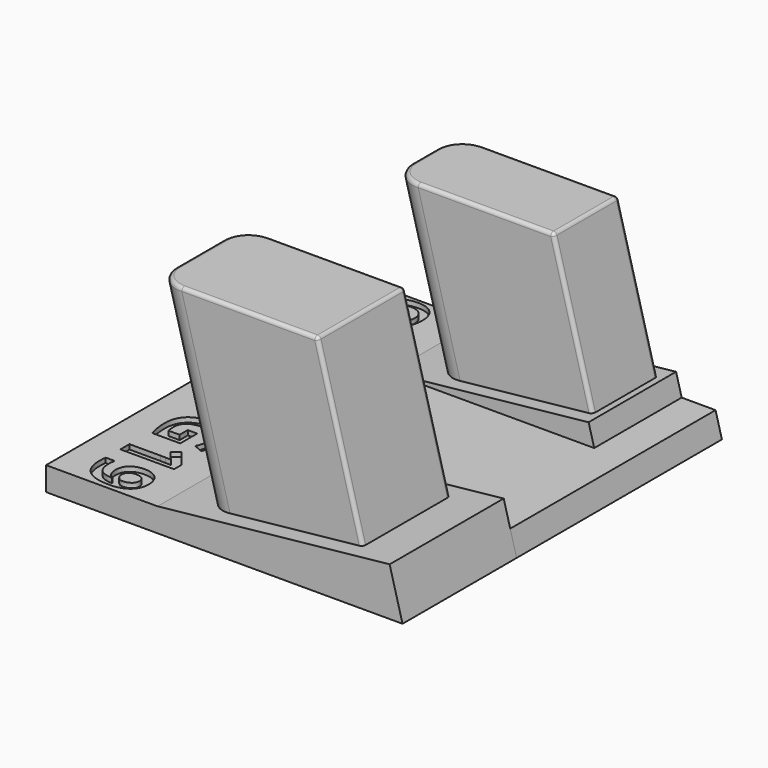
from build123d import *

# Parameters (mm, degrees)
F1_DEPTH        = 11.5
F3_DEPTH        = 15
F4_R            = 5.25
F6_DEPTH        = 84
F8_DEPTH        = 23
F11_DEPTH       = 8.575
F12_R           = 5.325
F14_DEPTH       = 23
F15_R           = 0.75
F16_TEXT_SIZE   = 12.157251404
F16_TEXT_SIZE_2 = 15.8246105662
F17_DEPTH       = 1


# Not quite as in the source:
# - Text() gives the source's letters only with a copy of the font that has no kerning and outlines rounded to 1/6400 em; it was checked with that copy


with BuildPart() as f1:
    # F0 (on Front) → F1 (new body, symmetric)
    with BuildSketch(Plane.XZ):
        Polygon((-29.1056600133, 44.8726974226), (-17.0820569768, 0), (17.0820569768, 0), (5.0584539402, 44.8726974226), align=None)
    extrude(amount=F1_DEPTH, both=True)

    # F2 (on Front) → F3 (join, symmetric)
    with BuildSketch(Plane.XZ):
        Polygon((25.7524949877, 0), (23.0374129665, 10.13282405), (-25.7981457243, 5), (-25.7981457243, 0), align=None)
    extrude(amount=F3_DEPTH, both=True)

    # F4
    f4_edges = [f1.edges().sort_by_distance(p)[0] for p in [
        (-23.864755, 11.5, 25.313373),
        (-23.864755, -11.5, 25.313373),
    ]]
    fillet(f4_edges, radius=F4_R)

    # F5 (on face) → F6 (join)
    with BuildSketch(Plane.XZ.offset(15)):
        Polygon((-49.2475050123, 0), (25.7524949877, 0), (24.4127490255, 5), (-49.2475050123, 5), align=None)
    extrude(amount=-F6_DEPTH)

    # F7 (on face) → F8 (join)
    with BuildSketch(Plane(origin=(0, 69, 0), x_dir=(-1, 0, 0), z_dir=(0, 1, 0))):
        Polygon((-23.0374129665, 10.13282405), (-25.7524949877, 0), (25.7981457243, 0), (25.7981457243, 5), align=None)
    extrude(amount=-F8_DEPTH)

    # F10 (on offset) → F11 (join, symmetric)
    with BuildSketch(Plane(origin=(0, 57.5, 0), x_dir=(-1, 0, 0), z_dir=(0, 1, 0))):
        Polygon((-6.3686802255, 39.9828663565), (-17.0820569768, 0), (17.0820569768, 0), (27.7954337281, 39.9828663565), align=None)
    extrude(amount=F11_DEPTH, both=True)

    # F12
    f12_edges = [f1.edges().sort_by_distance(p)[0] for p in [
        (-23.209642, 66.075, 22.868458),
        (-23.209642, 48.925, 22.868458),
    ]]
    fillet(f12_edges, radius=F12_R)

    # F13 (on face) + F8_face1 (on face) → F14 (cut, through all)
    with BuildSketch(Plane(origin=(0, 69, 0), x_dir=(-1, 0, 0), z_dir=(0, 1, 0))):
        Polygon((-17.2845549071, 5), (-16.1044685534, 9.4041422293), (-23.0374129665, 10.13282405), (-24.4127490255, 5), align=None)
    with BuildSketch(Plane(origin=(7.2173387559, 46, 6.71094135), x_dir=(-1, 0, 0), z_dir=(0, -1, 0))):
        Polygon((-15.8200742106, -3.4218827), (33.0154844802, 1.71094135), (-17.1954102697, 1.71094135), align=None)
    extrude(amount=-F14_DEPTH, dir=(0, 1, 0), mode=Mode.SUBTRACT)

    # F15
    f15_edges = [f1.edges().sort_by_distance(p)[0] for p in [
        (9.831461, -11.5, 27.059592),
        (9.831461, 11.5, 27.059592),
        (10.486574, 48.925, 24.614676),
        (10.486574, 66.075, 24.614676),
        (-7.956954, 48.925, 39.982866),
        (-26.146842, 50.452178, 39.982866),
        (6.36868, 57.5, 39.982866),
        (-27.795434, 57.5, 39.982866),
        (-7.956954, 66.075, 39.982866),
        (-26.146842, 64.547822, 39.982866),
        (-9.306003, 11.5, 44.872697),
        (-27.480288, 9.994331, 44.872697),
        (5.058454, 0, 44.872697),
        (-29.10566, 0, 44.872697),
        (-9.306003, -11.5, 44.872697),
        (-27.480288, -9.994331, 44.872697),
    ]]
    fillet(f15_edges, radius=F15_R)

    # F16 (on face) → F17 (cut)
    with BuildSketch(Plane.XY.offset(5)):
        with Locations(Location((-41.8994358738, 69), (0, 0, -90))):
            Text('G43', F16_TEXT_SIZE, font='Open Sans', font_style=FontStyle.BOLD, text_align=(TextAlign.LEFT, TextAlign.BOTTOM))
        with Locations(Location((-43.2196851722, 15), (0, 0, -90))):
            Text('G19', F16_TEXT_SIZE_2, font='Open Sans', font_style=FontStyle.BOLD, text_align=(TextAlign.LEFT, TextAlign.BOTTOM))
    extrude(amount=-F17_DEPTH, mode=Mode.SUBTRACT)


solid = f1.part
